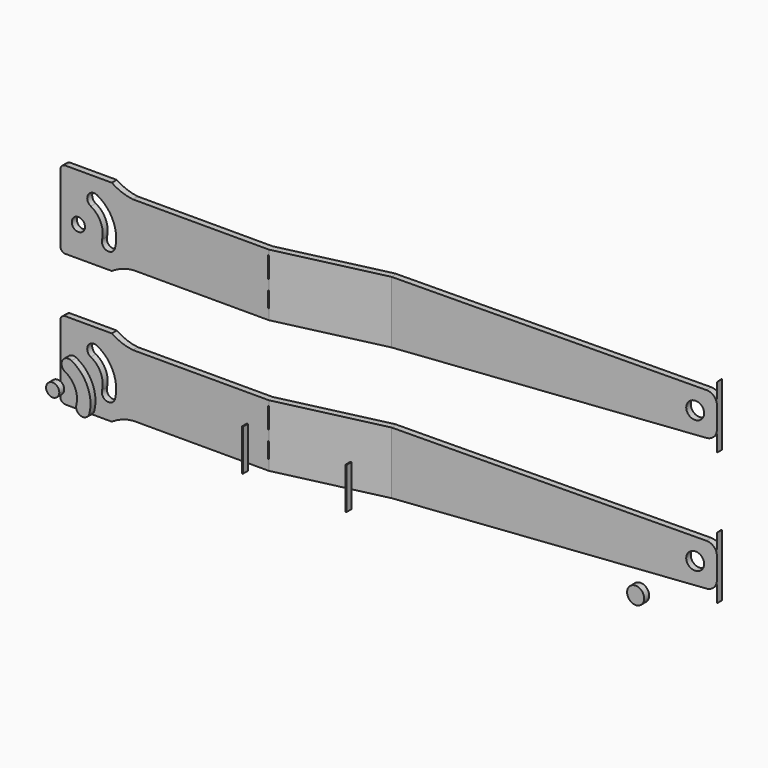
from build123d import *

# Parameters (mm, degrees)
F1_DEPTH  = 60
F3_R      = 8.25
F4_DEPTH  = 25
F5_DEPTH  = 6
F6_R      = 6.375
F7_DEPTH  = 25
F13_DEPTH = 6
F14_DEPTH = 25
F15_DEPTH = 25
F16_W     = 1
F16_H     = 20
F16_H_2   = 15
F17_DEPTH = 25
F20_R     = 6.375
F21_DEPTH = 6
F20_R_2   = 8.25
F20_W     = 1
F20_H     = 40
F23_DEPTH = 6


# Not quite as in the source:
# - a feature names something its author has since deleted; it is built from what else it names


with BuildPart() as f1:
    # F0 (on Top) → F1 (new body)
    with BuildSketch(Plane.XY):
        Polygon((-100, 0), (-300, 0), (-300, -6), (-98.6345753761, -6), align=None)
        Polygon((-0.3796555332, 22.9007694116), (-100, 0), (-98.6345753761, -6), (1.3654246239, 17), align=None)
        Polygon((300, 42.0855757845), (-0.3796555332, 22.9007694116), (1.3654246239, 17), (300, 36.0733506724), align=None)
    extrude(amount=F1_DEPTH)

    # F3 (on face) → F4 (cut)
    with BuildSketch(Plane(origin=(-1.0758067285, 16.8440821476, 0), x_dir=(0.9979666244, 0.0637386591, 0), z_dir=(0.0637386591, -0.9979666244, 0))):
        with BuildLine():
            Line((301.6892543085, 60), (2.4462054069, 60))
            Line((2.4462054069, 60), (292.0232443882, 50.3230153534))
            ThreePointArc((292.0232443882, 50.3230153534), (298.8774356083, 47.2805760816), (301.6892543085, 40.3285943784))
            Line((301.6892543085, 40.3285943784), (301.6892543085, 60))
        make_face()
        with BuildLine():
            Line((292.0232443882, 9.6769846466), (2.4462054069, 0))
            Line((2.4462054069, 0), (301.6892543085, 0))
            Line((301.6892543085, 0), (301.6892543085, 19.6714056216))
            ThreePointArc((301.6892543085, 19.6714056216), (298.8774356083, 12.7194239184), (292.0232443882, 9.6769846466))
        make_face()
        with Locations((281.6892543085, 30.0079316213)):
            Circle(F3_R)
    extrude(amount=-F4_DEPTH, mode=Mode.SUBTRACT)

    # F2 (on face) → F5 (join)
    with BuildSketch(Plane.XZ.offset(6)):
        with BuildLine():
            Line((-250.3, 67.5), (-295, 67.5))
            ThreePointArc((-295, 67.5), (-298.5355339059, 66.0355339059), (-300, 62.5))
            Line((-300, 62.5), (-300, 60))
            Line((-300, 60), (-230, 60))
            ThreePointArc((-230, 60), (-240.6075702178, 62.5115099439), (-250.3, 67.5))
        make_face()
    extrude(amount=-F5_DEPTH)

    # F6 (on face) → F7 (cut)
    with BuildSketch(Plane.XZ.offset(6)):
        with BuildLine():
            ThreePointArc((-259.7213383401, 16.1343621796), (-255.0196238496, 8.2353824448), (-247.1206441149, 12.9370969353))
            ThreePointArc((-247.1206441149, 12.9370969353), (-248.9955051627, 35.6089750865), (-264.4106548881, 52.339256668))
            ThreePointArc((-264.4106548881, 52.339256668), (-273.2189113282, 49.7096904517), (-270.5893451119, 40.9014340116))
            ThreePointArc((-270.5893451119, 40.9014340116), (-260.8998224273, 30.3852570175), (-259.7213383401, 16.1343621796))
        make_face()
        with Locations((-282.545583065, 21.5497146659)):
            Circle(F6_R)
    extrude(amount=-F7_DEPTH, mode=Mode.SUBTRACT)

    # F2 (on face) → F13 (join)
    with BuildSketch(Plane.XZ.offset(6)):
        with BuildLine():
            Line((-250.3, 67.5), (-295, 67.5))
            ThreePointArc((-295, 67.5), (-298.5355339059, 66.0355339059), (-300, 62.5))
            Line((-300, 62.5), (-300, 60))
            Line((-300, 60), (-300, 0))
            Line((-300, 0), (-300, -2.5))
            ThreePointArc((-300, -2.5), (-298.5355339059, -6.0355339059), (-295, -7.5))
            Line((-295, -7.5), (-250.3, -7.5))
            ThreePointArc((-250.3, -7.5), (-240.6075702178, -2.5115099439), (-230, 0))
            Line((-230, 0), (-230, 60))
            ThreePointArc((-230, 60), (-240.6075702178, 62.5115099439), (-250.3, 67.5))
        make_face()
    extrude(amount=-F13_DEPTH)

    # F6 (on face) → F14 (cut)
    with BuildSketch(Plane.XZ.offset(6)):
        with BuildLine():
            ThreePointArc((-259.7213383401, 16.1343621796), (-255.0196238496, 8.2353824448), (-247.1206441149, 12.9370969353))
            ThreePointArc((-247.1206441149, 12.9370969353), (-248.9955051627, 35.6089750865), (-264.4106548881, 52.339256668))
            ThreePointArc((-264.4106548881, 52.339256668), (-273.2189113282, 49.7096904517), (-270.5893451119, 40.9014340116))
            ThreePointArc((-270.5893451119, 40.9014340116), (-260.8998224273, 30.3852570175), (-259.7213383401, 16.1343621796))
        make_face()
        with Locations((-282.545583065, 21.5497146659)):
            Circle(F6_R)
    extrude(amount=-F14_DEPTH, mode=Mode.SUBTRACT)

    # F6 (on face) → F15 (cut)
    with BuildSketch(Plane.XZ.offset(6)):
        with BuildLine():
            ThreePointArc((-259.7213383401, 16.1343621796), (-255.0196238496, 8.2353824448), (-247.1206441149, 12.9370969353))
            ThreePointArc((-247.1206441149, 12.9370969353), (-248.9955051627, 35.6089750865), (-264.4106548881, 52.339256668))
            ThreePointArc((-264.4106548881, 52.339256668), (-273.2189113282, 49.7096904517), (-270.5893451119, 40.9014340116))
            ThreePointArc((-270.5893451119, 40.9014340116), (-260.8998224273, 30.3852570175), (-259.7213383401, 16.1343621796))
        make_face()
        with Locations((-282.545583065, 21.5497146659)):
            Circle(F6_R)
    extrude(amount=-F15_DEPTH, mode=Mode.SUBTRACT)

    # F16 (on face) → F17 (cut)
    with BuildSketch(Plane.XZ.offset(6)):
        with Locations((-99.1345753761, 45)):
            Rectangle(F16_W, F16_H)
        with Locations((-99.1345753761, 17.5)):
            Rectangle(F16_W, F16_H_2)
    extrude(amount=-F17_DEPTH, mode=Mode.SUBTRACT)


with BuildPart() as f18_1:
    # F18: copy of F1
    add(f1.part.moved(Location((0, 0, -128))))


with BuildPart() as f21:
    # F20 (on offset) → F21 (new body)
    with BuildSketch(Plane.XZ.offset(31)):
        with Locations((-282.545583065, -106.4502853341)):
            Circle(F20_R)
    extrude(amount=F21_DEPTH)


with BuildPart() as f21b:
    # F20 (on offset) → F21, piece 2 (new body)
    with BuildSketch(Plane.XZ.offset(31)):
        with BuildLine():
            ThreePointArc((-270.5893451119, -87.0985659884), (-260.8998224273, -97.6147429825), (-259.7213383401, -111.8656378204))
            ThreePointArc((-259.7213383401, -111.8656378204), (-255.0196238496, -119.7646175552), (-247.1206441149, -115.0629030647))
            ThreePointArc((-247.1206441149, -115.0629030647), (-248.9955051627, -92.3910249135), (-264.4106548881, -75.660743332))
            ThreePointArc((-264.4106548881, -75.660743332), (-273.2189113282, -78.2903095483), (-270.5893451119, -87.0985659884))
        make_face()
    extrude(amount=F21_DEPTH)


with BuildPart() as f21c:
    # F20 (on offset) → F21, piece 3 (new body)
    with BuildSketch(Plane.XZ.offset(31)):
        with Locations((280, -97.9920683787)):
            Circle(F20_R_2)
    extrude(amount=F21_DEPTH)


with BuildPart() as f21d:
    # F20 (on offset) → F21, piece 4 (new body)
    with BuildSketch(Plane.XZ.offset(31)):
        with Locations((-99.5, -98)):
            Rectangle(F20_W, F20_H)
    extrude(amount=F21_DEPTH)


with BuildPart() as f21e:
    # F20 (on offset) → F21, piece 5 (new body)
    with BuildSketch(Plane.XZ.offset(31)):
        with Locations((0.5, -98)):
            Rectangle(F20_W, F20_H)
    extrude(amount=F21_DEPTH)


with BuildPart() as f23:
    # F22 (on face) → F23 (new body)
    with BuildSketch(Plane.XY.offset(30)):
        with BuildLine():
            Line((-95.7337079203, 0.3963955631), (0, 22.4037032244))
            Line((0, 22.4037032244), (259.6203444668, 38.9852724063))
            Line((259.6203444668, 38.9852724063), (259.3428744797, 43.871647691))
            ThreePointArc((259.3428744797, 43.871647691), (254.3156644008, 54.2472956087), (243.4109197938, 57.9907506899))
            Line((243.4109197938, 57.9907506899), (-1.2747731814, 42.3630357116))
            ThreePointArc((-1.2747731814, 42.3630357116), (-2.8872435497, 42.1942015679), (-4.4807406449, 41.8953158635))
            Line((-4.4807406449, 41.8953158635), (-97.5157451123, 20.5083873609))
            ThreePointArc((-97.5157451123, 20.5083873609), (-99.741741069, 20.1275032673), (-101.9964857572, 20))
            Line((-101.9964857572, 20), (-217.4580631956, 20))
            ThreePointArc((-217.4580631956, 20), (-228.0646649134, 15.6066017178), (-232.4580631956, 5))
            Line((-232.4580631956, 5), (-232.4580631956, 0))
            Line((-232.4580631956, 0), (-100.7793098688, 0))
            Line((-100.7793098688, 0), (-100.1258566607, 0))
            Line((-100.1258566607, 0), (-95.7337079203, 0.3963955631))
        make_face()
    extrude(amount=F23_DEPTH)


solid = Compound([f1.part, f18_1.part, f21.part, f21b.part, f21c.part, f21d.part, f21e.part, f23.part])
